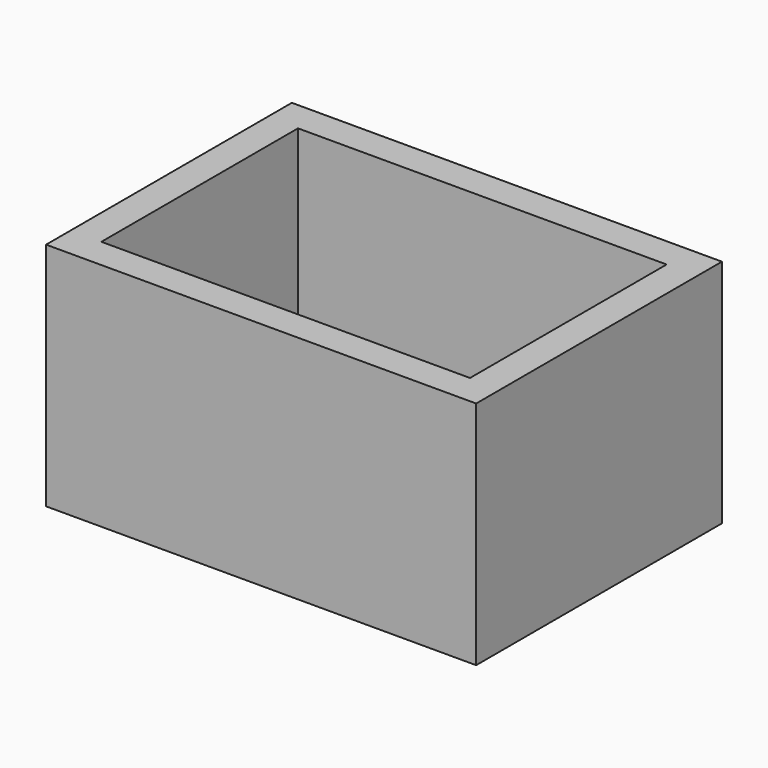
from build123d import *

# Parameters (mm, degrees)
F0_W     = 355.6
F0_H     = 254
F1_DEPTH = 190.5
F2_T     = -25.4
F4_D     = 5.08


with BuildPart() as f1:
    # F0 (on Top) → F1 (new body)
    with BuildSketch(Plane.XY):
        Rectangle(F0_W, F0_H)
    extrude(amount=F1_DEPTH)

    # F2
    f2_openings = [f1.faces().sort_by_distance(p)[0] for p in [
        (0, 0, 190.5),
    ]]
    offset(amount=F2_T, openings=f2_openings)

    # F4 (through all)
    with Locations(Plane.XY.offset(25.4)):
        with Locations((-127, 76.2), (-127, -76.2), (127, -76.2), (127, 76.2)):
            Hole(F4_D / 2)


solid = f1.part
